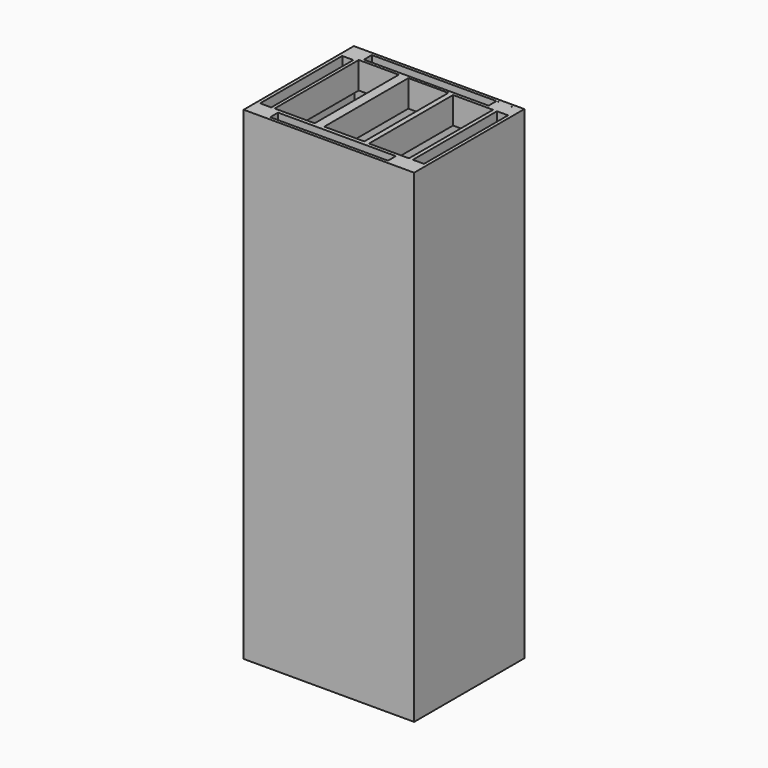
from build123d import *

# Parameters (mm, degrees)
F0_W     = 63.4695142508
F0_H     = 51.2949377298
F0_W_2   = 61
F0_H_2   = 49
F1_DEPTH = 180
F3_W     = 2.2321660072
F3_H     = 3.732714802
F3_W_2   = 14.8959429935
F3_H_2   = 39.1232501715
F3_W_3   = 3.5938005894
F3_H_3   = 1.2999996543
F3_W_4   = 1.4519924298
F4_DEPTH = 10


# Not quite as in the source:
# - a feature names something its author has since deleted; it is built from what else it names
# - the program builds the solid bodies; features that only make, move or delete a surface that nothing else refers to are left out


with BuildPart() as f1:
    # F0 (on Top) → F1 (new body)
    with BuildSketch(Plane.XY):
        Rectangle(F0_W, F0_H)
        Rectangle(F0_W_2, F0_H_2, mode=Mode.SUBTRACT)
    extrude(amount=-F1_DEPTH)

    # F3 (on Top) → F4 (join)
    with BuildSketch(Plane.XY):
        with Locations((-25.2534588799, 22.6865075529)):
            Rectangle(F3_W, F3_H)
        Polygon((-24.1373758763, 20.8201501518), (-26.3695418835, 20.8201501518), (-26.3695418835, 18.7030434608), (-26.3695418835, -19.5201504976), (-22.775741294, -19.5201504976), (-22.775741294, -20.8201501518), (21.0672114044, -20.8201501518), (21.0672114044, -19.5201504976), (10.0216064602, -19.5201504976), (10.0216064602, 19.603099674), (22.2738981247, 19.603099674), (22.2738981247, 20.8201501518), align=None)
        with Locations((-17.7230439149, 0.1456094906)):
            Rectangle(F3_W_2, F3_H_2, mode=Mode.SUBTRACT)
        with Locations((0.6728977896, 0.226427801)):
            Rectangle(F3_W_2, F3_H_2, mode=Mode.SUBTRACT)
        Polygon((-26.3695418835, 18.7030434608), (-26.3695418835, 20.8201501518), (-26.3695418835, 24.5528649539), (-30.5465664715, 24.5528649539), (-30.5465664715, 18.7030434608), align=None)
        Polygon((22.2738981247, 24.4889948517), (22.2738981247, 20.8201501518), (26.3695418835, 20.8201501518), (26.3695418835, 19.603099674), (30.5195916444, 19.603099674), (30.5195916444, 24.4889948517), align=None)
        Polygon((26.3695418835, 20.8201501518), (22.2738981247, 20.8201501518), (22.2738981247, 19.603099674), (24.9175494537, 19.603099674), (26.3695418835, 19.603099674), align=None)
        with Locations((-24.5726415887, -20.1701503247)):
            Rectangle(F3_W_3, F3_H_3)
        Polygon((-26.3695418835, -20.8201501518), (-26.3695418835, -19.5201504976), (-30.8873578906, -19.5201504976), (-30.8873578906, -24.8510874808), (-22.775741294, -24.8510874808), (-22.775741294, -20.8201501518), align=None)
        with Locations((25.6435456686, 0.0414745882)):
            Rectangle(F3_W_4, F3_H_2)
        Polygon((31.1229377985, -19.5201504976), (26.3695418835, -19.5201504976), (26.3695418835, -20.8201501518), (21.0672114044, -20.8201501518), (21.0672114044, -24.8510874808), (31.1229377985, -24.8510874808), align=None)
        Polygon((26.3695418835, -20.8201501518), (26.3695418835, -19.5201504976), (24.9175494537, -19.5201504976), (21.0672114044, -19.5201504976), (21.0672114044, -20.8201501518), align=None)
    extrude(amount=-F4_DEPTH)


solid = f1.part
